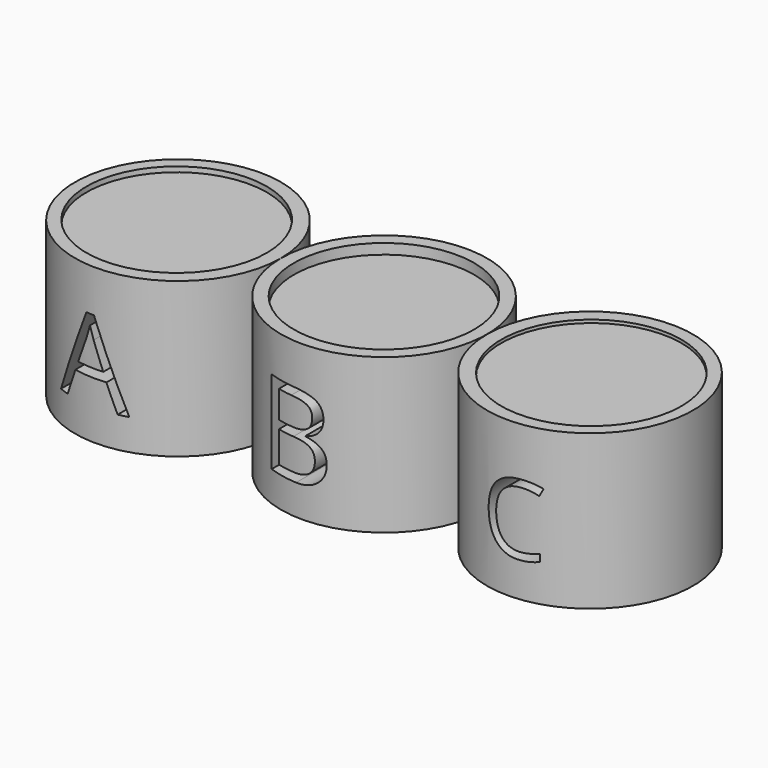
from build123d import *

# Parameters (mm, degrees)
F0_R           = 25.4
F1_DEPTH       = 38.1
F4_TEXT_SIZE   = 27.9099861574
F4_TEXT_SIZE_2 = 28.8452450063
F4_TEXT_SIZE_3 = 23.9790003333
F5_DEPTH       = 12.7
F2_R           = 22.219427589
F6_DEPTH       = 1.27
F2_R_2         = 22.2268245579
F7_DEPTH       = 2.54
F2_R_3         = 22.2207835739
F8_DEPTH       = 0.762


# Not quite as in the source:
# - Text() gives the source's letters only with a copy of the font that has no kerning and outlines rounded to 1/6400 em; it was checked with that copy


with BuildPart() as f1:
    # F0 (on Top) → F1 (new body)
    with BuildSketch(Plane.XY):
        with Locations((-58.3538132187, 0)):
            Circle(F0_R)
    extrude(amount=F1_DEPTH)


with BuildPart() as f1b:
    # F0 (on Top) → F1, piece 2 (new body)
    with BuildSketch(Plane.XY):
        with BuildLine():
            ThreePointArc((68.6461867813, 0), (43.2461867813, 25.4), (17.8461867813, 0))
            ThreePointArc((17.8461867813, 0), (43.2461867813, -25.4), (68.6461867813, 0))
        make_face()
    extrude(amount=F1_DEPTH)


with BuildPart() as f1c:
    # F0 (on Top) → F1, piece 3 (new body)
    with BuildSketch(Plane.XY):
        with BuildLine():
            ThreePointArc((17.8461867813, 0), (-7.5538132187, 25.4), (-32.9538132187, 0))
            ThreePointArc((-32.9538132187, 0), (-7.5538132187, -25.4), (17.8461867813, 0))
        make_face()
    extrude(amount=F1_DEPTH)


with BuildPart() as f5_tool:
    # F4 (on offset) → F5 (new body)
    with BuildSketch(Plane.XZ.offset(25.4)):
        with Locations((-68.5846507549, 7.6360823587)):
            Text('A', F4_TEXT_SIZE, font='Open Sans', text_align=(TextAlign.LEFT, TextAlign.BOTTOM))
        with Locations((-18.9702556612, 7.5059629013)):
            Text('B', F4_TEXT_SIZE_2, font='Open Sans', text_align=(TextAlign.LEFT, TextAlign.BOTTOM))
        with Locations((36.7028266191, 8.7682045996)):
            Text('C', F4_TEXT_SIZE_3, font='Open Sans', text_align=(TextAlign.LEFT, TextAlign.BOTTOM))
    extrude(amount=-F5_DEPTH)


with BuildPart() as f1_1:
    add(f1.part)

    # F5: cut by f5_tool
    add(f5_tool.part, mode=Mode.SUBTRACT)

    # F2 (on face) → F6 (cut)
    with BuildSketch(Plane.XY.offset(38.1)):
        with Locations((-58.6840132187, 0)):
            Circle(F2_R)
    extrude(amount=-F6_DEPTH, mode=Mode.SUBTRACT)


with BuildPart() as f1b_1:
    add(f1b.part)

    # F5: cut by f5_tool
    add(f5_tool.part, mode=Mode.SUBTRACT)

    # F2 (on face) → F8 (cut)
    with BuildSketch(Plane.XY.offset(38.1)):
        with Locations((43.5763867813, 0)):
            Circle(F2_R_3)
    extrude(amount=-F8_DEPTH, mode=Mode.SUBTRACT)


with BuildPart() as f1c_1:
    add(f1c.part)

    # F5: cut by f5_tool
    add(f5_tool.part, mode=Mode.SUBTRACT)

    # F2 (on face) → F7 (cut)
    with BuildSketch(Plane.XY.offset(38.1)):
        with Locations((-7.5538132187, 0)):
            Circle(F2_R_2)
    extrude(amount=-F7_DEPTH, mode=Mode.SUBTRACT)


solid = Compound([f1_1.part, f1b_1.part, f1c_1.part])
